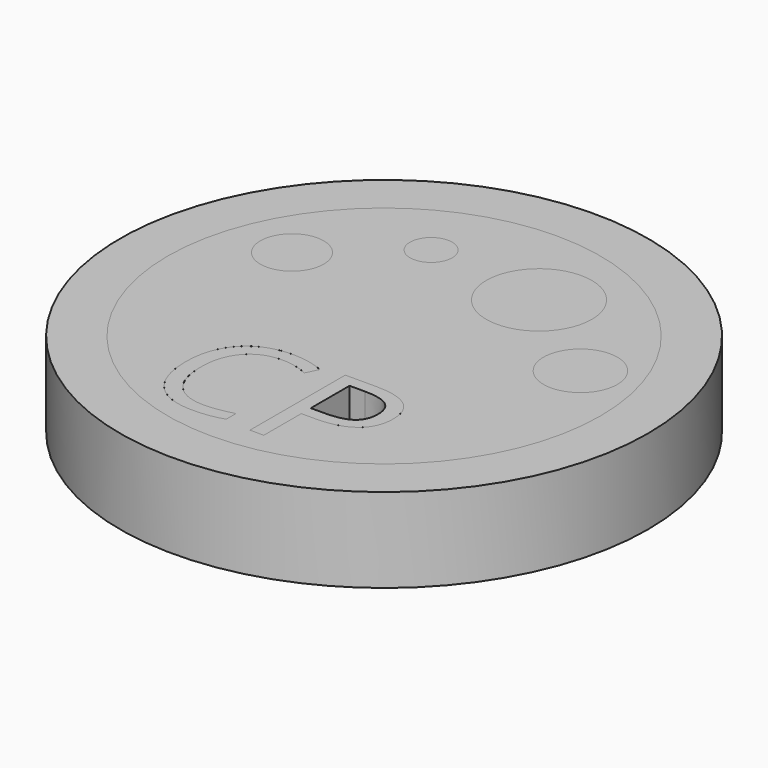
from build123d import *

# Parameters (mm, degrees)
F0_R         = 25
F0_R_2       = 20.5
F1_DEPTH     = 8
F0_R_3       = 3
F0_R_4       = 2
F0_R_5       = 5
F0_R_6       = 3.5
F2_DEPTH     = 3
F0_TEXT_SIZE = 15.814672488
F3_DEPTH     = 8
F4_DEPTH     = 3
F5_DEPTH     = 5


# Not quite as in the source:
# - Text() gives the source's letters only with a copy of the font that has no kerning and outlines rounded to 1/6400 em; it was checked with that copy


with BuildPart() as f1:
    # F0 (on Top) → F1 (new body)
    with BuildSketch(Plane.XY):
        Circle(F0_R)
        Circle(F0_R_2, mode=Mode.SUBTRACT)
    extrude(amount=F1_DEPTH)

    # F0 (on Top) → F2 (join)
    with BuildSketch(Plane.XY):
        Circle(F0_R_2)
        with BuildLine():
            add(Edge.make_bspline(
                [(-0.9068726255, -8.2980953516), (-2.1893437226, -7.6976320056), (-3.4718148196, -7.6976320056)],
                knots=[0, 0, 0, 1, 1, 1], degree=2))
            add(Edge.make_bspline(
                [(-3.4718148196, -7.6976320056), (-5.3325098795, -7.6976320056), (-6.4098844428, -8.9368598576)],
                knots=[0, 0, 0, 1, 1, 1], degree=2))
            add(Edge.make_bspline(
                [(-6.4098844428, -8.9368598576), (-7.487259006, -10.1760877096), (-7.487259006, -12.330836836)],
                knots=[0, 0, 0, 1, 1, 1], degree=2))
            add(Edge.make_bspline(
                [(-7.487259006, -12.330836836), (-7.487259006, -14.5448909844), (-6.4481856027, -15.7544663254)],
                knots=[0, 0, 0, 1, 1, 1], degree=2))
            add(Edge.make_bspline(
                [(-6.4481856027, -15.7544663254), (-5.4091121994, -16.9640416665), (-3.4866410751, -16.9640416665)],
                knots=[0, 0, 0, 1, 1, 1], degree=2))
            add(Edge.make_bspline(
                [(-3.4866410751, -16.9640416665), (-2.3054827236, -16.9640416665), (-0.7907336244, -16.5390223434)],
                knots=[0, 0, 0, 1, 1, 1], degree=2))
            Line((-0.7907336244, -16.5390223434), (-0.7907336244, -17.6880571413))
            add(Edge.make_bspline(
                [(-0.7907336244, -17.6880571413), (-1.9644788481, -18.1303737625), (-3.6867955238, -18.1303737625)],
                knots=[0, 0, 0, 1, 1, 1], degree=2))
            add(Edge.make_bspline(
                [(-3.6867955238, -18.1303737625), (-6.1800774832, -18.1303737625), (-7.5354443363, -16.6156246633)],
                knots=[0, 0, 0, 1, 1, 1], degree=2))
            add(Edge.make_bspline(
                [(-7.5354443363, -16.6156246633), (-8.8908111893, -15.100875564), (-8.8908111893, -12.313539538)],
                knots=[0, 0, 0, 1, 1, 1], degree=2))
            add(Edge.make_bspline(
                [(-8.8908111893, -12.313539538), (-8.8908111893, -10.5689834792), (-8.2384559492, -9.2568598712)],
                knots=[0, 0, 0, 1, 1, 1], degree=2))
            add(Edge.make_bspline(
                [(-8.2384559492, -9.2568598712), (-7.5861007091, -7.9447362632), (-6.3542859848, -7.2343115225)],
                knots=[0, 0, 0, 1, 1, 1], degree=2))
            add(Edge.make_bspline(
                [(-6.3542859848, -7.2343115225), (-5.1224712606, -6.5238867819), (-3.4545175216, -6.5238867819)],
                knots=[0, 0, 0, 1, 1, 1], degree=2))
            add(Edge.make_bspline(
                [(-3.4545175216, -6.5238867819), (-1.6803089518, -6.5238867819), (-0.3508880458, -7.1712999368)],
                knots=[0, 0, 0, 1, 1, 1], degree=2))
            Line((-0.3508880458, -7.1712999368), (-0.9068726255, -8.2980953516))
        make_face(mode=Mode.SUBTRACT)
        with BuildLine():
            add(Edge.make_bspline(
                [(4.601081277, -6.6845045493), (8.8315061675, -6.6845045493), (8.8315061675, -9.9734622183)],
                knots=[0, 0, 0, 1, 1, 1], degree=2))
            add(Edge.make_bspline(
                [(8.8315061675, -9.9734622183), (8.8315061675, -11.6883657662), (7.6614675077, -12.6113001684)],
                knots=[0, 0, 0, 1, 1, 1], degree=2))
            add(Edge.make_bspline(
                [(7.6614675077, -12.6113001684), (6.4914288478, -13.5342345707), (4.3144403381, -13.5342345707)],
                knots=[0, 0, 0, 1, 1, 1], degree=2))
            Line((4.3144403381, -13.5342345707), (2.9850194321, -13.5342345707))
            Line((2.9850194321, -13.5342345707), (2.9850194321, -17.9746980802))
            Line((2.9850194321, -17.9746980802), (1.6728958241, -17.9746980802))
            Line((1.6728958241, -17.9746980802), (1.6728958241, -6.6845045493))
            Line((1.6728958241, -6.6845045493), (4.601081277, -6.6845045493))
        make_face(mode=Mode.SUBTRACT)
        with Locations((-13.6713000034, 6.1915926617)):
            Circle(F0_R_3, mode=Mode.SUBTRACT)
        with Locations((-5.8897417039, 12.9314828664)):
            Circle(F0_R_4, mode=Mode.SUBTRACT)
        with Locations((5.3362494572, 11.6726538104)):
            Circle(F0_R_5, mode=Mode.SUBTRACT)
        with Locations((14.8226446854, 4.719500086)):
            Circle(F0_R_6, mode=Mode.SUBTRACT)
    extrude(amount=F2_DEPTH)

    # F0 (on Top) → F3 (join)
    with BuildSketch(Plane.XY):
        with Locations((-9.8569888367, -17.9746980802)):
            Text('CP', F0_TEXT_SIZE, font='Open Sans', text_align=(TextAlign.LEFT, TextAlign.BOTTOM))
        with Locations((-13.6713000034, 6.1915926617)):
            Circle(F0_R_3)
        with Locations((-5.8897417039, 12.9314828664)):
            Circle(F0_R_4)
        with Locations((5.3362494572, 11.6726538104)):
            Circle(F0_R_5)
        with Locations((14.8226446854, 4.719500086)):
            Circle(F0_R_6)
    extrude(amount=F3_DEPTH)

    # F0 (on Top) → F4 (join)
    with BuildSketch(Plane.XY):
        with BuildLine():
            Line((2.9850194321, -7.8211841344), (2.9850194321, -12.4074391559))
            Line((2.9850194321, -12.4074391559), (4.1686488261, -12.4074391559))
            add(Edge.make_bspline(
                [(4.1686488261, -12.4074391559), (5.913204885, -12.4074391559), (6.6928188178, -11.8440414485)],
                knots=[0, 0, 0, 1, 1, 1], degree=2))
            add(Edge.make_bspline(
                [(6.6928188178, -11.8440414485), (7.4724327506, -11.2806437411), (7.4724327506, -10.0352382827)],
                knots=[0, 0, 0, 1, 1, 1], degree=2))
            add(Edge.make_bspline(
                [(7.4724327506, -10.0352382827), (7.4724327506, -8.9158559957), (6.7385331054, -8.368520065)],
                knots=[0, 0, 0, 1, 1, 1], degree=2))
            add(Edge.make_bspline(
                [(6.7385331054, -8.368520065), (6.0046334603, -7.8211841344), (4.4528187224, -7.8211841344)],
                knots=[0, 0, 0, 1, 1, 1], degree=2))
            Line((4.4528187224, -7.8211841344), (2.9850194321, -7.8211841344))
        make_face()
    extrude(amount=F4_DEPTH)


with BuildPart() as f5:
    # F5 (new): a face of the model
    f5_faces = [f1.part.faces().sort_by_distance(p)[0] for p in [
        (-0.5598248639, -0.5199803208, 3),
    ]]
    extrude(f5_faces, amount=F5_DEPTH)


solid = Compound([f1.part, f5.part])
